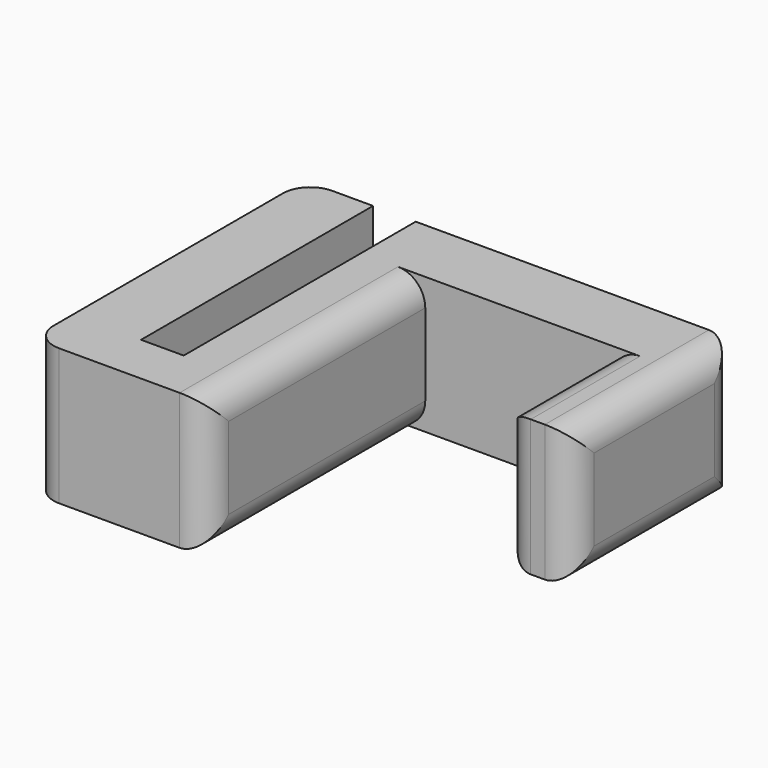
from build123d import *

# Parameters (mm, degrees)
F1_DEPTH     = 25.4
F2_R         = 5.08
F3_TEXT_SIZE = 19.772476258
F4_DEPTH     = 3


# Not quite as in the source:
# - Text() gives the source's letters only with a copy of the font that has no kerning and outlines rounded to 1/6400 em; it was checked with that copy


with BuildPart() as f1:
    # F0 (on Top) → F1 (new body)
    with BuildSketch(Plane.XY):
        Polygon((0, 63.5), (0, 0), (32.5752518936, 0), (32.5752518936, 50.8), (67.4797778515, 50.8), (67.4797778515, 25.3516854542), (80.2734648196, 25.3516854542), (80.2734648196, 63.5), (20.6375, 63.5), (20.6375, 9.52754), (12.7, 9.52754), (12.7, 63.5), align=None)
    extrude(amount=F1_DEPTH)

    # F2
    f2_edges = [f1.edges().sort_by_distance(p)[0] for p in [
        (80.273465, 63.5, 12.7),
        (80.273465, 25.351685, 12.7),
        (67.479778, 25.351685, 12.7),
        (32.575252, 0, 12.7),
        (0, 0, 12.7),
        (0, 63.5, 12.7),
        (32.575252, 25.4, 25.4),
        (67.479778, 38.075843, 25.4),
        (80.273465, 44.425843, 25.4),
        (80.273465, 44.425843, 0),
        (67.479778, 38.075843, 0),
        (32.575252, 25.4, 0),
    ]]
    fillet(f2_edges, radius=F2_R)

    # F3 (on face) → F4 (join)
    with BuildSketch(Plane(origin=(0, 0, 0), x_dir=(0, -1, 0), z_dir=(-1, 0, 0))):
        with Locations((-55.9856947511, 5.5073467083)):
            Text('WILL', F3_TEXT_SIZE, font='Open Sans', font_style=FontStyle.BOLD, text_align=(TextAlign.LEFT, TextAlign.BOTTOM))
    extrude(amount=F4_DEPTH)


solid = f1.part
